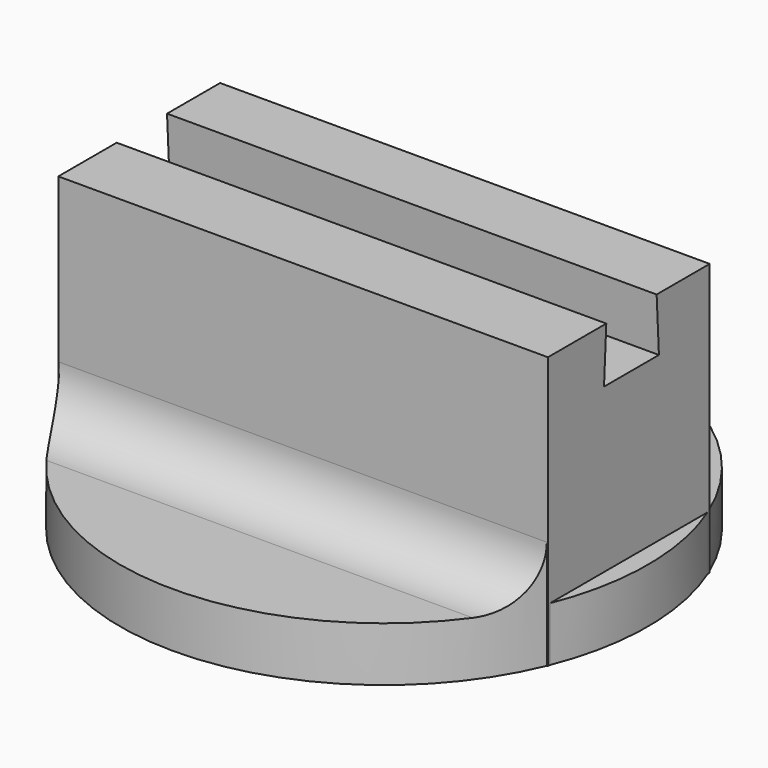
from build123d import *

# Parameters (mm, degrees)
F0_R        = 24.2537643176
F1_DEPTH    = 5
F2_W        = 45.0000017881
F2_H        = 18.5869578272
F3_DEPTH    = 25
F4_W        = 45.0000017881
F4_H        = 5.7842824608
F5_DEPTH    = 5
F6_DEPTH    = 5
F6_TAPER    = -3
F7_DEPTH    = 5
F7_TAPER    = -3
F8_R        = 5
F9_T4_DEPTH = 43.1102228968
F9_S5_R     = 24.2537643176
F9_T6_DEPTH = 23


# Not quite as in the source:
# - a fillet or chamfer that OpenCascade refuses, or shapes differently, is made with other operations: its cross-section is extruded or revolved along the edge and cut away or added


with BuildPart() as f1:
    # F0 (on Top) → F1 (new body)
    with BuildSketch(Plane.XY):
        Circle(F0_R)
    extrude(amount=F1_DEPTH)

    # F2 (on Top) → F3 (join)
    with BuildSketch(Plane.XY):
        Rectangle(F2_W, F2_H)
    extrude(amount=F3_DEPTH)

    # F4 (on face) → F5 (join)
    with BuildSketch(Plane.XY.offset(25)):
        with Locations((0, 0.3060454037)):
            Rectangle(F4_W, F4_H)
    extrude(amount=-F5_DEPTH)

    # F4 (on face) → F6 (join)
    with BuildSketch(Plane.XY.offset(25)):
        with Locations((0, 0.3060454037)):
            Rectangle(F4_W, F4_H)
    extrude(amount=-F6_DEPTH, taper=F6_TAPER)

    # F4 (on face) → F7 (cut)
    with BuildSketch(Plane.XY.offset(25)):
        with Locations((0, 0.3060454037)):
            Rectangle(F4_W, F4_H)
    extrude(amount=-F7_DEPTH, taper=F7_TAPER, mode=Mode.SUBTRACT)

    # F8
    f8_edges = [f1.edges().sort_by_distance(p)[0] for p in [
        (0, -9.293479, 5),
    ]]
    fillet(f8_edges, radius=F8_R)

    # F9: fillet of radius 5 on 1 edges, made by hand


with BuildPart() as f9_tool2:
    # F9_s3 → F9_t4 (new body)
    with BuildSketch(Plane.XZ.offset(21.5551114484)):
        with BuildLine():
            ThreePointArc((-22.5000008941, 10), (-23.9644669881, 6.4644660941), (-27.5000008941, 5))
            Line((-27.5000008941, 5), (-22.5000008941, 5))
            Line((-22.5000008941, 5), (-22.5000008941, 10))
        make_face()
    extrude(amount=-F9_T4_DEPTH)

    # F9_s5 → F9_t6 (intersect, symmetric)
    with BuildSketch(Plane.XY.offset(7.5)):
        Circle(F9_S5_R)
    extrude(amount=F9_T6_DEPTH, both=True, mode=Mode.INTERSECT)


with BuildPart() as f1_1:
    add(f1.part)

    # F9_t1: union F9_tool2
    add(f9_tool2.part)


solid = f1_1.part
